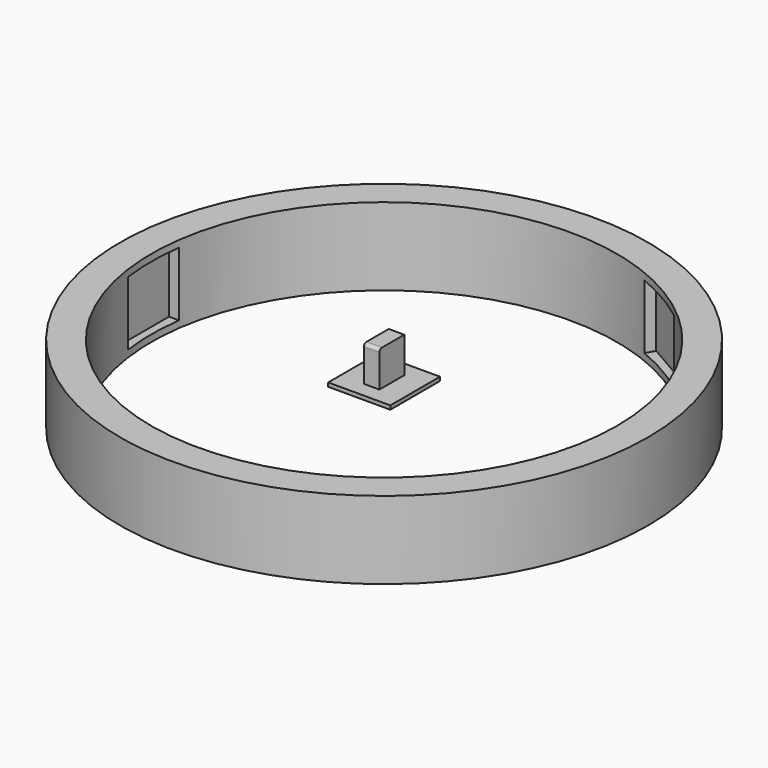
from build123d import *

# Parameters (mm, degrees)
F0_R            = 431.8
F0_R_2          = 381
F1_DEPTH        = 63.5
F2_W            = 50.8
F2_H            = 104.775
F3_DEPTH        = 52.3875
F3_COPIES_COUNT = 3
F4_W            = 101.6
F4_H            = 101.6
F5_DEPTH        = 6.35
F6_W            = 25.4
F6_H            = 50.8
F7_DEPTH        = 58.42
F8_R            = 5.08


# Not quite as in the source:
# - a pattern or mirror of a feature is missing from the dataset's text; its kind, count and spacing are read off the source's solid


with BuildPart() as f1:
    # F0 (on Top) → F1 (new body, symmetric)
    with BuildSketch(Plane.XY):
        Circle(F0_R)
        Circle(F0_R_2, mode=Mode.SUBTRACT)
    extrude(amount=F1_DEPTH, both=True)

    # F2 (on Front) → F3 (cut, symmetric)
    with BuildSketch(Plane.XZ):
        with Locations((-368.3, 0)):
            Rectangle(F2_W, F2_H)
    f3 = extrude(amount=F3_DEPTH, both=True, mode=Mode.SUBTRACT)

    # F3_copies: F3 ×3 about axis
    f3_copies_axis = Axis((0, 0, 0), (0, 0, 1))
    for i in range(1, F3_COPIES_COUNT):
        add(f3.rotate(f3_copies_axis, i * 360 / F3_COPIES_COUNT), mode=Mode.SUBTRACT)


with BuildPart() as f5:
    # F4 (on Top) → F5 (new body)
    with BuildSketch(Plane.XY):
        Rectangle(F4_W, F4_H)
    extrude(amount=F5_DEPTH)

    # F6 (on face) → F7 (join)
    with BuildSketch(Plane.XY.offset(6.35)):
        Rectangle(F6_W, F6_H)
    extrude(amount=F7_DEPTH)

    # F8
    f8_edges = [f5.edges().sort_by_distance(p)[0] for p in [
        (0, -25.4, 64.77),
    ]]
    fillet(f8_edges, radius=F8_R)


solid = Compound([f1.part, f5.part])
